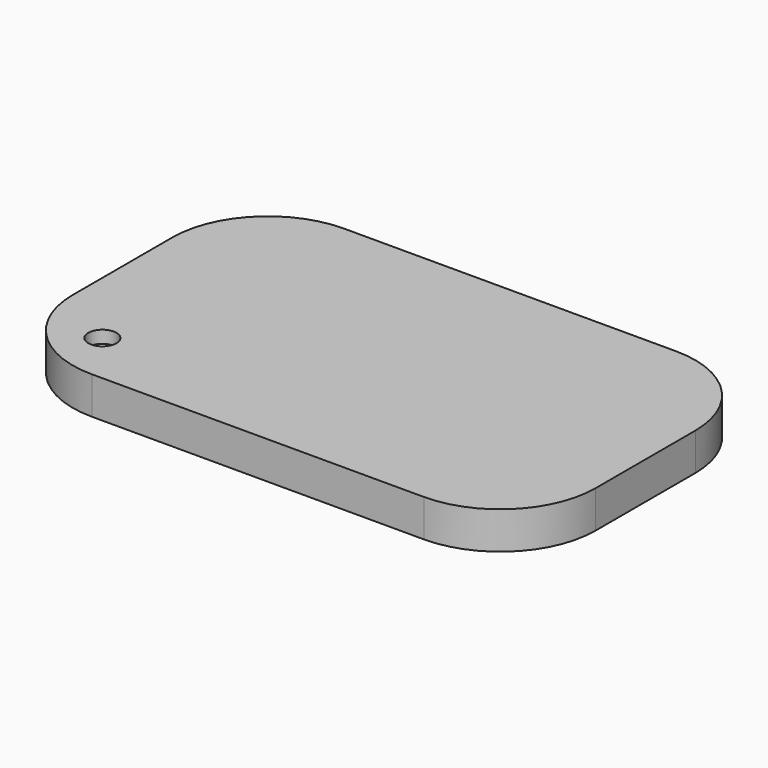
from build123d import *

# Parameters (mm, degrees)
F0_W         = 60
F0_H         = 35
F1_DEPTH     = 3
F2_R         = 10
F3_T         = 1.5
F4_TEXT_SIZE = 11.1111111111
F5_DEPTH     = 1.5
F7_D         = 3.4


# Not quite as in the source:
# - Text() gives the source's letters only with a copy of the font that has no kerning and outlines rounded to 1/6400 em; it was checked with that copy


with BuildPart() as f1:
    # F0 (on Top) → F1 (new body)
    with BuildSketch(Plane.XY):
        Rectangle(F0_W, F0_H)
    extrude(amount=F1_DEPTH)

    # F2
    f2_edges = [f1.edges().sort_by_distance(p)[0] for p in [
        (30, 17.5, 1.5),
        (-30, -17.5, 1.5),
        (30, -17.5, 1.5),
        (-30, 17.5, 1.5),
    ]]
    fillet(f2_edges, radius=F2_R)

    # F3
    f3_openings = [f1.faces().sort_by_distance(p)[0] for p in [
        (0, 0, 0),
    ]]
    offset(amount=F3_T, openings=f3_openings, kind=Kind.INTERSECTION)

    # F4 (on face) → F5 (join)
    with BuildSketch(Plane(origin=(0, 0, 3), x_dir=(1, 0, 0), z_dir=(0, 0, -1))):
        with Locations((-26.7558911176, -3.6342963271)):
            Text('TC Gossau', F4_TEXT_SIZE, font='Open Sans', text_align=(TextAlign.LEFT, TextAlign.BOTTOM))
    extrude(amount=F5_DEPTH)

    # F7 (through all)
    with Locations(Plane(origin=(0, 0, 3), x_dir=(1, 0, 0), z_dir=(0, 0, -1))):
        with Locations((-23.8400995731, 12.6071702689)):
            Hole(F7_D / 2)


solid = f1.part
